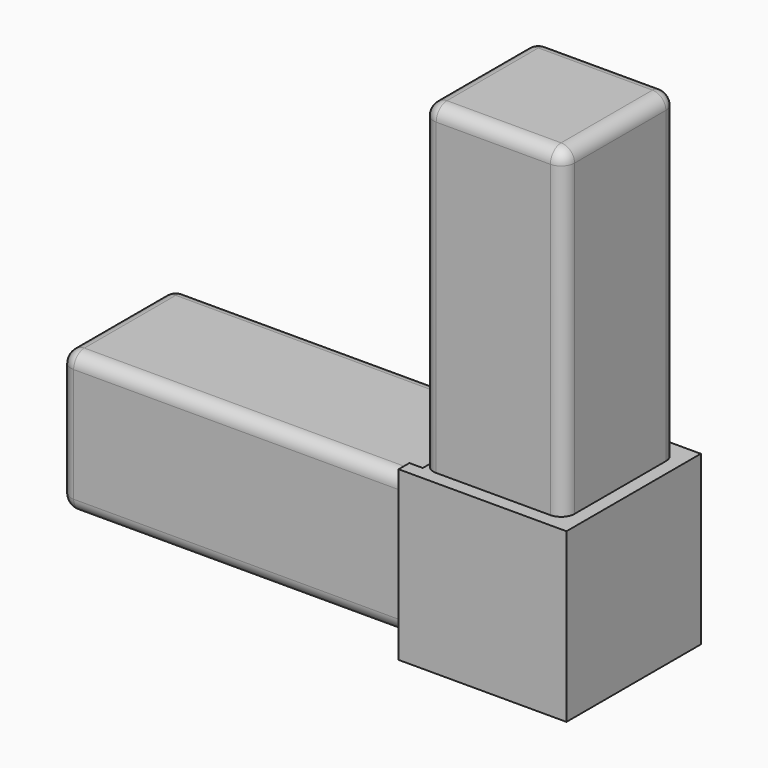
from build123d import *

# Parameters (mm, degrees)
F0_W     = 21
F0_H     = 48
F0_W_2   = 52
F0_H_2   = 21
F1_DEPTH = 21
F0_W_3   = 2
F0_H_3   = 2
F2_DEPTH = 2
F3_W     = 25
F3_H     = 25
F4_DEPTH = 2
F5_W     = 25
F5_H     = 25
F6_DEPTH = 2
F7_W     = 25
F7_H     = 25
F8_DEPTH = 2
F9_R     = 2


with BuildPart() as f1:
    # F0 (on Front) → F1 (new body)
    with BuildSketch(Plane.XZ):
        with Locations((27, 36.5)):
            Rectangle(F0_W, F0_H)
        with Locations((-11.5, 0)):
            Rectangle(F0_W_2, F0_H_2)
        Polygon((14.5, -10.5), (37.5, -10.5), (37.5, 10.5), (37.5, 12.5), (16.5, 12.5), (16.5, 10.5), (14.5, 10.5), align=None)
    extrude(amount=F1_DEPTH)

    # F0 (on Front) → F2 (join)
    with BuildSketch(Plane.XZ):
        Polygon((37.5, 10.5), (37.5, -10.5), (14.5, -10.5), (14.5, -12.5), (39.5, -12.5), (39.5, 12.5), (37.5, 12.5), align=None)
        with Locations((15.5, 11.5)):
            Rectangle(F0_W_3, F0_H_3)
        Polygon((14.5, -10.5), (37.5, -10.5), (37.5, 10.5), (37.5, 12.5), (16.5, 12.5), (16.5, 10.5), (14.5, 10.5), align=None)
    extrude(amount=-F2_DEPTH)

    # F3 (on face) → F4 (join)
    with BuildSketch(Plane.XZ.offset(21)):
        with Locations((27, 0)):
            Rectangle(F3_W, F3_H)
    extrude(amount=F4_DEPTH)

    # F5 (on face) → F6 (join)
    with BuildSketch(Plane.YZ.offset(37.5)):
        with Locations((-10.5, 0)):
            Rectangle(F5_W, F5_H)
    extrude(amount=F6_DEPTH)

    # F7 (on face) → F8 (join)
    with BuildSketch(Plane(origin=(0, 0, -10.5), x_dir=(1, 0, 0), z_dir=(0, 0, -1))):
        with Locations((27, 10.5)):
            Rectangle(F7_W, F7_H)
    extrude(amount=F8_DEPTH)

    # F9
    f9_edges = [f1.edges().sort_by_distance(p)[0] for p in [
        (-37.5, -10.5, -10.5),
        (-37.5, 0, 0),
        (-37.5, -10.5, 10.5),
        (-37.5, -21, 0),
        (27, 0, 60.5),
        (16.5, -10.5, 60.5),
        (37.5, -10.5, 60.5),
        (27, -21, 60.5),
        (16.5, -21, 36.5),
        (37.5, -21, 36.5),
        (37.5, 0, 36.5),
        (16.5, 0, 36.5),
        (-11.5, 0, 10.5),
        (-11.5, 0, -10.5),
        (-11.5, -21, 10.5),
        (-11.5, -21, -10.5),
    ]]
    fillet(f9_edges, radius=F9_R)


solid = f1.part
